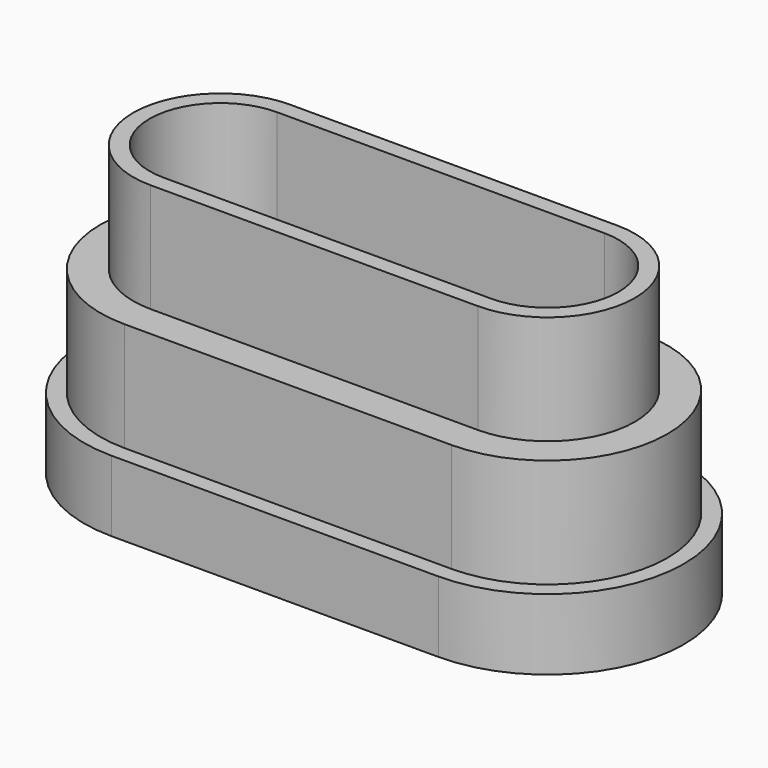
from build123d import *

# Parameters (mm, degrees)
F1_DEPTH      = 3
F2_DEPTH      = 10
F4_DEPTH      = 20
F4_DEPTH_BACK = 2
F6_DEPTH      = 20
F6_DEPTH_BACK = 2
F7_DEPTH      = 2


with BuildPart() as f1:
    # F0 (on Top) → F1 (new body)
    with BuildSketch(Plane.XY):
        with BuildLine():
            Line((30, 25), (-30, 25))
            ThreePointArc((-30, 25), (-55, 0), (-30, -25))
            Line((-30, -25), (30, -25))
            ThreePointArc((30, -25), (55, 0), (30, 25))
        make_face()
        with BuildLine():
            ThreePointArc((-30, -22.0000010729), (-52.0000010729, 0), (-30, 22.0000010729))
            Line((-30, 22.0000010729), (30, 22.0000010729))
            ThreePointArc((30, 22.0000010729), (52.0000010729, 0), (30, -22.0000010729))
            Line((30, -22.0000010729), (-30, -22.0000010729))
        make_face(mode=Mode.SUBTRACT)
        with BuildLine():
            Line((30, 22.0000010729), (-30, 22.0000010729))
            ThreePointArc((-30, 22.0000010729), (-52.0000010729, 0), (-30, -22.0000010729))
            Line((-30, -22.0000010729), (30, -22.0000010729))
            ThreePointArc((30, -22.0000010729), (52.0000010729, 0), (30, 22.0000010729))
        make_face()
    extrude(amount=-F1_DEPTH)

    # F0 (on Top) → F2 (join)
    with BuildSketch(Plane.XY):
        with BuildLine():
            Line((30, 25), (-30, 25))
            ThreePointArc((-30, 25), (-55, 0), (-30, -25))
            Line((-30, -25), (30, -25))
            ThreePointArc((30, -25), (55, 0), (30, 25))
        make_face()
        with BuildLine():
            ThreePointArc((-30, -22.0000010729), (-52.0000010729, 0), (-30, 22.0000010729))
            Line((-30, 22.0000010729), (30, 22.0000010729))
            ThreePointArc((30, 22.0000010729), (52.0000010729, 0), (30, -22.0000010729))
            Line((30, -22.0000010729), (-30, -22.0000010729))
        make_face(mode=Mode.SUBTRACT)
    extrude(amount=F2_DEPTH)


with BuildPart() as f4:
    # F3 (on face) → F4 (new body, two sides)
    with BuildSketch(Plane.XY.offset(10)) as f4_sk:
        with BuildLine():
            Line((30, 22.0000010729), (-30, 22.0000010729))
            ThreePointArc((-30, 22.0000010729), (-52.0000010729, 0), (-30, -22.0000010729))
            Line((-30, -22.0000010729), (30, -22.0000010729))
            ThreePointArc((30, -22.0000010729), (52.0000010729, 0), (30, 22.0000010729))
        make_face()
        with BuildLine():
            ThreePointArc((-30, -19.0000024438), (-49.0000024438, 0), (-30, 19.0000024438))
            Line((-30, 19.0000024438), (30, 19.0000024438))
            ThreePointArc((30, 19.0000024438), (49.0000024438, 0), (30, -19.0000024438))
            Line((30, -19.0000024438), (-30, -19.0000024438))
        make_face(mode=Mode.SUBTRACT)
    extrude(amount=F4_DEPTH)
    extrude(f4_sk.sketch, amount=-F4_DEPTH_BACK)

    # F5 (on face) → F7 (join)
    with BuildSketch(Plane.XY.offset(30)):
        with BuildLine():
            Line((30, 19.0000024438), (-30, 19.0000024438))
            ThreePointArc((-30, 19.0000024438), (-49.0000024438, 0), (-30, -19.0000024438))
            Line((-30, -19.0000024438), (30, -19.0000024438))
            ThreePointArc((30, -19.0000024438), (49.0000024438, 0), (30, 19.0000024438))
        make_face()
        with BuildLine():
            ThreePointArc((-30, -16.0000026226), (-46.0000026226, 0), (-30, 16.0000026226))
            Line((-30, 16.0000026226), (30, 16.0000026226))
            ThreePointArc((30, 16.0000026226), (46.0000026226, 0), (30, -16.0000026226))
            Line((30, -16.0000026226), (-30, -16.0000026226))
        make_face(mode=Mode.SUBTRACT)
    extrude(amount=-F7_DEPTH)


with BuildPart() as f6:
    # F5 (on face) → F6 (new body, two sides)
    with BuildSketch(Plane.XY.offset(30)) as f6_sk:
        with BuildLine():
            Line((30, 16.0000026226), (-30, 16.0000026226))
            ThreePointArc((-30, 16.0000026226), (-46.0000026226, 0), (-30, -16.0000026226))
            Line((-30, -16.0000026226), (30, -16.0000026226))
            ThreePointArc((30, -16.0000026226), (46.0000026226, 0), (30, 16.0000026226))
        make_face()
        with BuildLine():
            ThreePointArc((-30, -13.0000026226), (-43.0000026226, 0), (-30, 13.0000026226))
            Line((-30, 13.0000026226), (30, 13.0000026226))
            ThreePointArc((30, 13.0000026226), (43.0000026226, 0), (30, -13.0000026226))
            Line((30, -13.0000026226), (-30, -13.0000026226))
        make_face(mode=Mode.SUBTRACT)
    extrude(amount=F6_DEPTH)
    extrude(f6_sk.sketch, amount=-F6_DEPTH_BACK)


solid = Compound([f1.part, f4.part, f6.part])
